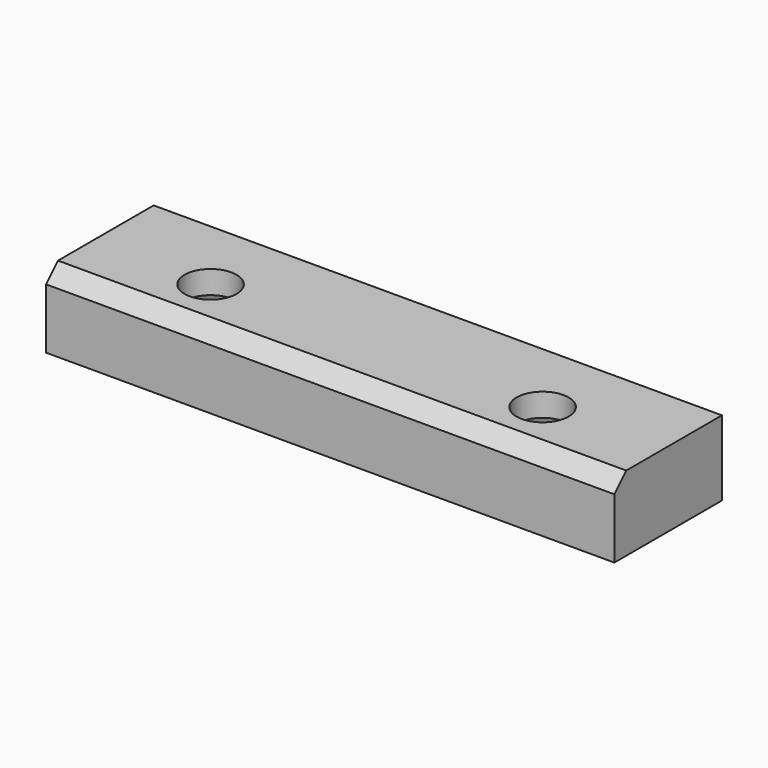
from build123d import *

# Parameters (mm, degrees)
F0_W     = 76.5
F0_H     = 18.1
F0_R     = 3.5
F1_DEPTH = 10.1
F2_R     = 5.5
F3_DEPTH = 7
F4_R     = 1.99999
F5_SIZE  = 2


# Not quite as in the source:
# - a fillet or chamfer is up to 0.001 mm smaller than in the source, because OpenCascade refuses the exact size
# - a feature names something its author has since deleted; it is built from what else it names


with BuildPart() as f1:
    # F0 (on Top) → F1 (new body)
    with BuildSketch(Plane.XY):
        with Locations((38.25, -9.05)):
            Rectangle(F0_W, F0_H)
        with Locations((15.9, -10.3)):
            Circle(F0_R, mode=Mode.SUBTRACT)
        with Locations((60.6, -10.3)):
            Circle(F0_R, mode=Mode.SUBTRACT)
    extrude(amount=F1_DEPTH)

    # F2 (on face) → F3 (cut)
    with BuildSketch(Plane(origin=(0, 0, 0), x_dir=(1, 0, 0), z_dir=(0, 0, -1))):
        with Locations((60.6, 10.3)):
            Circle(F2_R)
        with Locations((15.9, 10.3)):
            Circle(F2_R)
    extrude(amount=-F3_DEPTH, mode=Mode.SUBTRACT)

    # F4 (radius 2 in the source; OpenCascade refuses exactly that, so slightly less here)
    f4_edges = [f1.edges().sort_by_distance(p)[0] for p in [
        (55.1, -10.3, 7),
        (10.4, -10.3, 7),
    ]]
    fillet(f4_edges, radius=F4_R)

    # F5
    f5_edges = [f1.edges().sort_by_distance(p)[0] for p in [
        (38.25, -18.1, 10.1),
    ]]
    chamfer(f5_edges, length=F5_SIZE)


solid = f1.part
